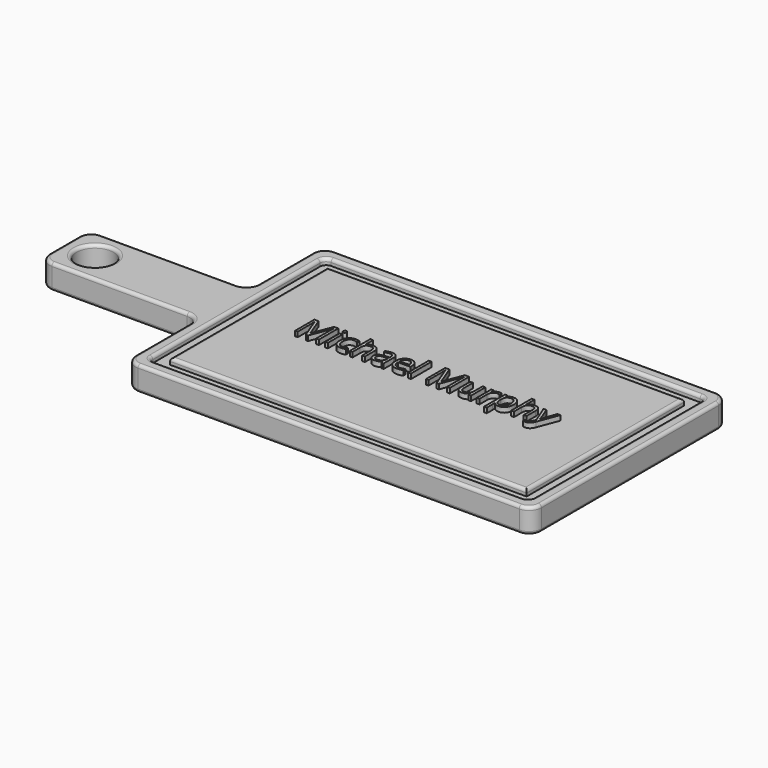
from build123d import *

# Parameters (mm, degrees)
F0_W         = 165.1
F0_H         = 63.5
F1_DEPTH     = 25.4
F2_R         = 19.05
F3_DEPTH     = 25.4
F5_DEPTH     = 6.35
F6_R         = 6.35
F7_R         = 12.7
F8_R         = 3.175
F9_TEXT_SIZE = 34.8672684696
F10_DEPTH    = 5.08


# Not quite as in the source:
# - Text() gives the source's letters only with a copy of the font that has no kerning and outlines rounded to 1/6400 em; it was checked with that copy


with BuildPart() as f1:
    # F0 (on Top) → F1 (new body)
    with BuildSketch(Plane.XY):
        Polygon((0, 95.25), (0, 0), (419.1, 0), (419.1, 254), (0, 254), (0, 158.75), align=None)
        with Locations((-82.55, 127)):
            Rectangle(F0_W, F0_H)
    extrude(amount=-F1_DEPTH)

    # F2 (on Top) → F3 (cut)
    with BuildSketch(Plane.XY):
        with Locations((-133.35, 127)):
            Circle(F2_R)
    extrude(amount=-F3_DEPTH, mode=Mode.SUBTRACT)

    # F4 (on face) → F5 (cut)
    with BuildSketch(Plane.XY):
        Polygon((12.6999982595, 95.25), (12.6999982595, 12.6999982595), (406.4000017405, 12.6999982595), (406.4000017405, 241.3000017405), (12.6999982595, 241.3000017405), (12.6999982595, 158.75), align=None)
        Polygon((25.4000046253, 95.25), (25.4000046253, 158.75), (25.4000046253, 228.5999953747), (393.6999953747, 228.5999953747), (393.6999953747, 25.4000046253), (25.4000046253, 25.4000046253), align=None, mode=Mode.SUBTRACT)
    extrude(amount=-F5_DEPTH, mode=Mode.SUBTRACT)

    # F6
    f6_edges = [f1.edges().sort_by_distance(p)[0] for p in [
        (12.699998, 241.300002, -3.175),
        (406.400002, 12.699998, -3.175),
        (12.699998, 12.699998, -3.175),
        (406.400002, 241.300002, -3.175),
    ]]
    fillet(f6_edges, radius=F6_R)

    # F7
    f7_edges = [f1.edges().sort_by_distance(p)[0] for p in [
        (0, 0, -12.7),
        (-165.1, 95.25, -12.7),
        (-165.1, 158.75, -12.7),
        (0, 158.75, -12.7),
        (0, 254, -12.7),
        (419.1, 254, -12.7),
        (419.1, 0, -12.7),
        (0, 95.25, -12.7),
    ]]
    fillet(f7_edges, radius=F7_R)

    # F8
    f8_edges = [f1.edges().sort_by_distance(p)[0] for p in [
        (209.55, 228.599995, 0),
        (393.699995, 127, 0),
        (209.55, 25.400005, 0),
        (25.400005, 127, 0),
        (0, 47.625, -25.4),
        (-3.719744, 91.530256, -25.4),
        (3.719744, 3.719744, -25.4),
        (-82.55, 95.25, -25.4),
        (209.55, 0, -25.4),
        (-161.380256, 98.969744, -25.4),
        (415.380256, 3.719744, -25.4),
        (-165.1, 127, -25.4),
        (419.1, 127, -25.4),
        (-161.380256, 155.030256, -25.4),
        (415.380256, 250.280256, -25.4),
        (-82.55, 158.75, -25.4),
        (209.55, 254, -25.4),
        (-3.719744, 162.469744, -25.4),
        (3.719744, 250.280256, -25.4),
        (0, 206.375, -25.4),
        (-152.4, 127, -25.4),
        (0, 47.625, 0),
        (-3.719744, 91.530256, 0),
        (3.719744, 3.719744, 0),
        (-82.55, 95.25, 0),
        (209.55, 0, 0),
        (-161.380256, 98.969744, 0),
        (415.380256, 3.719744, 0),
        (-165.1, 127, 0),
        (419.1, 127, 0),
        (-161.380256, 155.030256, 0),
        (415.380256, 250.280256, 0),
        (-82.55, 158.75, 0),
        (209.55, 254, 0),
        (-3.719744, 162.469744, 0),
        (3.719744, 250.280256, 0),
        (0, 206.375, 0),
        (209.55, 12.699998, 0),
        (14.55987, 14.55987, 0),
        (404.54013, 14.55987, 0),
        (12.699998, 127, 0),
        (406.400002, 127, 0),
        (14.55987, 239.44013, 0),
        (404.54013, 239.44013, 0),
        (209.55, 241.300002, 0),
        (-152.4, 127, 0),
    ]]
    fillet(f8_edges, radius=F8_R)

    # F9 (on Top) → F10 (join)
    with BuildSketch(Plane.XY):
        with Locations((77.2740263492, 117.7438050508)):
            Text('Michael Murphy', F9_TEXT_SIZE, font='Open Sans', text_align=(TextAlign.LEFT, TextAlign.BOTTOM))
    extrude(amount=F10_DEPTH)


solid = f1.part
